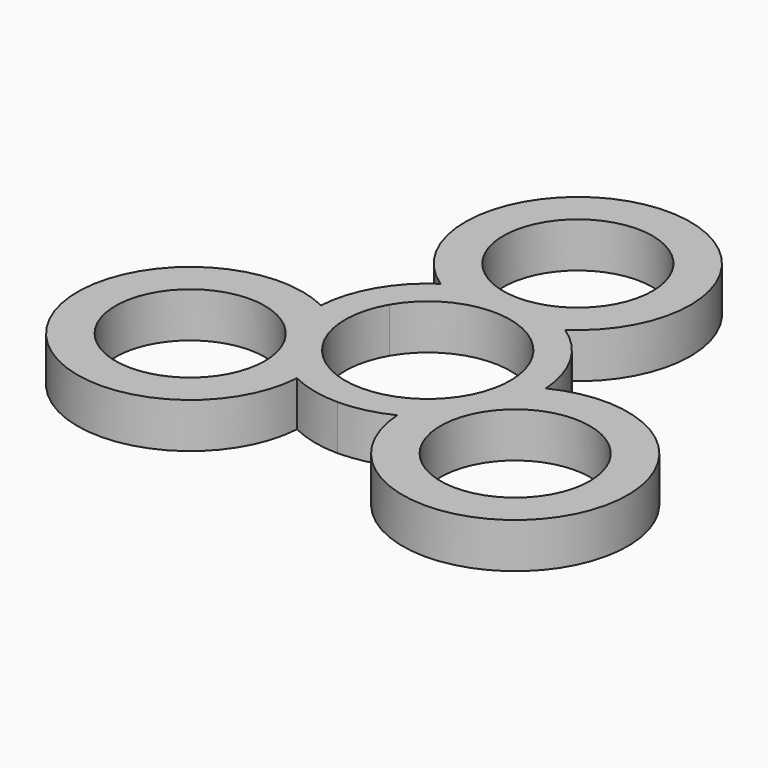
from build123d import *

# Parameters (mm, degrees)
F0_R     = 9.95
F1_DEPTH = 6


# Not quite as in the source:
# - a feature names something its author has since deleted; it is built from what else it names


with BuildPart() as f1:
    # F0 (on Top) → F1 (new body)
    with BuildSketch(Plane.XY):
        with BuildLine():
            ThreePointArc((8.2915619759, 12.5), (0, 40), (-8.2915619759, 12.5))
            ThreePointArc((-8.2915619759, 12.5), (-10.9307033082, 10.2722794544), (-12.9903810568, 7.5))
            ThreePointArc((-12.9903810568, 7.5), (-14.3614066163, 4.3301270189), (-14.9710985352, 0.9307033082))
            ThreePointArc((-14.9710985352, 0.9307033082), (-34.6410161514, -20), (-6.6795365594, -13.4307033082))
            ThreePointArc((-6.6795365594, -13.4307033082), (-3.4307033082, -14.6024064733), (0, -15))
            ThreePointArc((0, -15), (3.4307033082, -14.6024064733), (6.6795365594, -13.4307033082))
            ThreePointArc((6.6795365594, -13.4307033082), (34.6410161514, -20), (14.9710985352, 0.9307033082))
            ThreePointArc((14.9710985352, 0.9307033082), (14.3614066163, 4.3301270189), (12.9903810568, 7.5))
            ThreePointArc((12.9903810568, 7.5), (10.9307033082, 10.2722794544), (8.2915619759, 12.5))
        make_face()
        with Locations((-21.6506350946, -12.5)):
            Circle(F0_R, mode=Mode.SUBTRACT)
        with Locations((21.6506350946, -12.5)):
            Circle(F0_R, mode=Mode.SUBTRACT)
        with BuildLine():
            ThreePointArc((-9.5262794416, 5.5), (0, 11), (9.5262794416, 5.5))
            ThreePointArc((9.5262794416, 5.5), (9.5262794416, -5.5), (0, -11))
            ThreePointArc((0, -11), (-9.5262794416, -5.5), (-9.5262794416, 5.5))
        make_face(mode=Mode.SUBTRACT)
        with Locations((0, 25)):
            Circle(F0_R, mode=Mode.SUBTRACT)
    extrude(amount=-F1_DEPTH)


solid = f1.part
